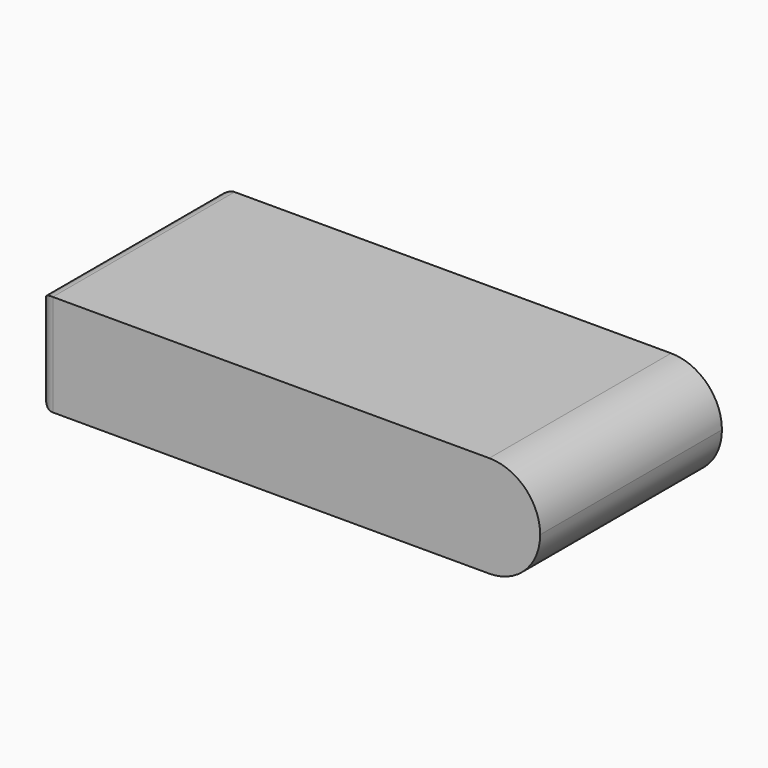
from build123d import *

# Parameters (mm, degrees)
F0_W     = 71.5
F0_H     = 32.4
F1_DEPTH = 14.5
F2_R     = 2
F3_R     = 7.24999


# Not quite as in the source:
# - a fillet or chamfer is up to 0.001 mm smaller than in the source, because OpenCascade refuses the exact size


with BuildPart() as f1:
    # F0 (on Top) → F1 (new body)
    with BuildSketch(Plane.XY):
        Rectangle(F0_W, F0_H)
    extrude(amount=F1_DEPTH)

    # F2
    f2_edges = [f1.edges().sort_by_distance(p)[0] for p in [
        (-35.75, 16.2, 7.25),
        (-35.75, -16.2, 7.25),
        (-35.75, 0, 0),
        (-35.75, 0, 14.5),
    ]]
    fillet(f2_edges, radius=F2_R)

    # F3 (radius 7.25 in the source; OpenCascade refuses exactly that, so slightly less here)
    f3_edges = [f1.edges().sort_by_distance(p)[0] for p in [
        (35.75, 0, 14.5),
        (35.75, 0, 0),
    ]]
    fillet(f3_edges, radius=F3_R)


solid = f1.part
